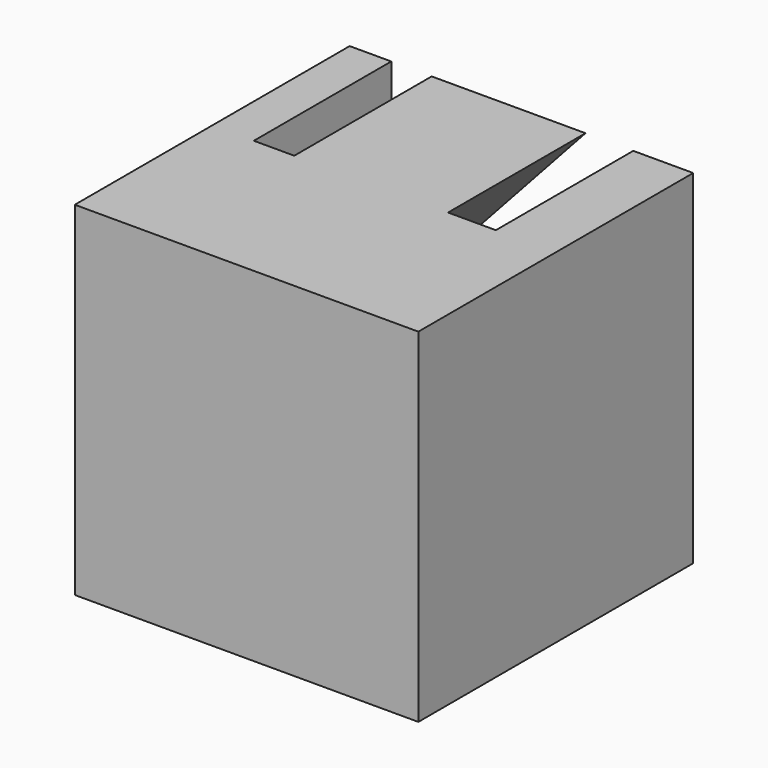
from build123d import *

# Parameters (mm, degrees)
F0_W         = 10
F0_H         = 10
F1_DEPTH     = 10
F2_TEXT_SIZE = 14.1858550099
F3_DEPTH     = 25.4


# Not quite as in the source:
# - Text() gives the source's letters only with a copy of the font that has no kerning and outlines rounded to 1/6400 em; it was checked with that copy


with BuildPart() as f1:
    # F0 (on Top) → F1 (new body)
    with BuildSketch(Plane.XY):
        Rectangle(F0_W, F0_H)
    extrude(amount=F1_DEPTH)

    # F2 (on Front) → F3 (cut)
    with BuildSketch(Plane.XZ):
        with Locations((-5.1809209399, 0)):
            Text('K', F2_TEXT_SIZE, font='Open Sans', text_align=(TextAlign.LEFT, TextAlign.BOTTOM))
    extrude(amount=-F3_DEPTH, mode=Mode.SUBTRACT)


solid = f1.part
